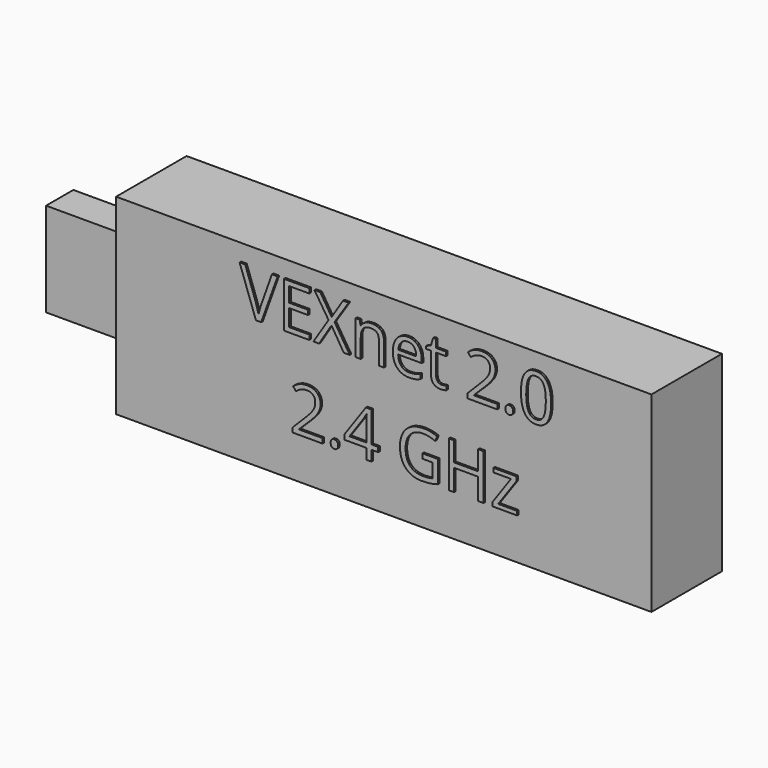
from build123d import *

# Parameters (mm, degrees)
F1_DEPTH     = 5.6769
F0_W         = 11.811
F0_H         = 12.1158
F2_DEPTH     = 2.1971
F3_TEXT_SIZE = 8.2366090889
F4_DEPTH     = 0.254


# Not quite as in the source:
# - Text() gives the source's letters only with a copy of the font that has no kerning and outlines rounded to 1/6400 em; it was checked with that copy


with BuildPart() as f1:
    # F0 (on Front) → F1 (new body, symmetric)
    with BuildSketch(Plane.XZ):
        Polygon((26.9971612774, 12.2625256074), (-42.0146387226, 12.2625256074), (-42.0146387226, 5.9887256074), (-42.0146387226, -6.1270743926), (-42.0146387226, -12.4262743926), (26.9971612774, -12.4262743926), align=None)
    extrude(amount=F1_DEPTH, both=True)

    # F0 (on Front) → F2 (join, symmetric)
    with BuildSketch(Plane.XZ):
        with Locations((-47.9201387226, -0.0691743926)):
            Rectangle(F0_W, F0_H)
    extrude(amount=F2_DEPTH, both=True)


with BuildPart() as f4:
    # F3 (on face) → F4 (new body)
    with BuildSketch(Plane.XZ.offset(5.6769)):
        with Locations((-25.8941805223, 4.2663030326)):
            Text('VEXnet 2.0', F3_TEXT_SIZE, font='Open Sans', text_align=(TextAlign.LEFT, TextAlign.BOTTOM))
        with Locations((-19.4734863435, -6.9354853282)):
            Text('2.4 GHz', F3_TEXT_SIZE, font='Open Sans', text_align=(TextAlign.LEFT, TextAlign.BOTTOM))
    extrude(amount=F4_DEPTH)


solid = Compound([f1.part, f4.part])
